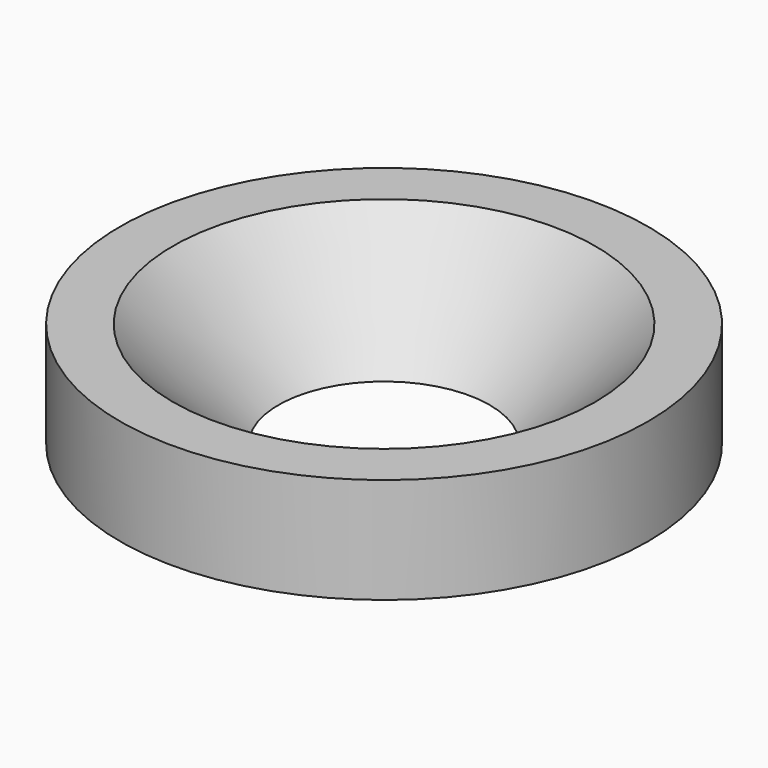
from build123d import *

# Parameters (mm, degrees)
F0_R     = 12.5
F0_R_2   = 5
F1_DEPTH = 5
F2_SIZE  = 4.99999


# Not quite as in the source:
# - a fillet or chamfer is up to 0.001 mm smaller than in the source, because OpenCascade refuses the exact size


with BuildPart() as f1:
    # F0 (on Top) → F1 (new body)
    with BuildSketch(Plane.XY):
        Circle(F0_R)
        Circle(F0_R_2, mode=Mode.SUBTRACT)
    extrude(amount=F1_DEPTH)

    # F2 (size 5 in the source; OpenCascade refuses exactly that, so slightly less here)
    f2_edges = [f1.edges().sort_by_distance(p)[0] for p in [
        (-5, 0, 5),
    ]]
    chamfer(f2_edges, length=F2_SIZE)


solid = f1.part
